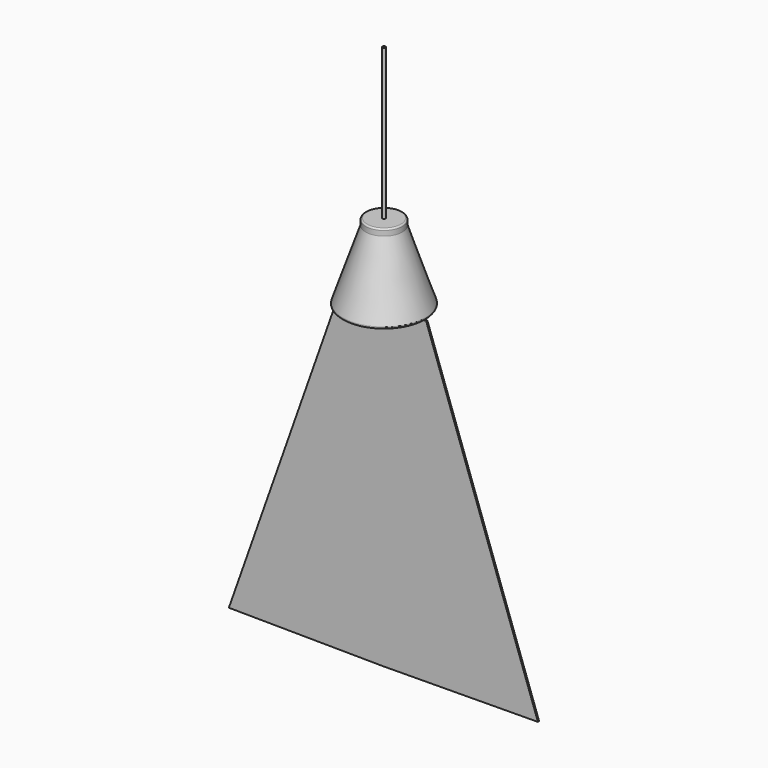
from build123d import *

# Parameters (mm, degrees)
F2_T     = -2
F3_R     = 3
F4_DEPTH = 300
F6_DEPTH = 1.5


# Not quite as in the source:
# - a shell that OpenCascade refuses in one call is made with other operations: the cavity is built on its own and cut out


with BuildPart() as f1:
    # F0 (on Front) → F1 (revolve)
    with BuildSketch(Plane.XZ):
        with BuildLine():
            Line((33.5040265024, 286.039857173), (0, 286.039857173))
            Line((0, 286.039857173), (0, 133.639857173))
            Line((0, 133.639857173), (79.491585897, 133.639857173))
            ThreePointArc((79.491585897, 133.639857173), (81.9292301706, 134.8911746988), (82.33336311, 137.6012635761))
            Line((82.33336311, 137.6012635761), (36.5040265024, 273.0661034584))
            Line((36.5040265024, 273.0661034584), (36.5040265024, 283.039857173))
            ThreePointArc((36.5040265024, 283.039857173), (35.6253468459, 285.1611775165), (33.5040265024, 286.039857173))
        make_face()
    revolve(axis=Axis((0, 0, 248.212441802), (0, 0, 1)))

    # F2: a shell. OpenCascade refuses it in one call, so the cavity is built on its own and cut out:
    # the body offset inwards by the wall thickness, plus a prism from it out through each open face.
    f2_core = offset(f1.part, amount=F2_T, kind=Kind.INTERSECTION, mode=Mode.PRIVATE)
    f2_exits = [f2_core.faces().sort_by_distance(p)[0] for p in [
        (0, 0, 135.639857),
    ]]
    add(f2_core, mode=Mode.SUBTRACT)
    extrude(f2_exits, amount=-F2_T, mode=Mode.SUBTRACT)

    # F3 (on face) → F4 (join)
    with BuildSketch(Plane.XY.offset(286.039857173)):
        Circle(F3_R)
    extrude(amount=F4_DEPTH)

    # F5 (on Front) → F6 (join, symmetric)
    with BuildSketch(Plane.XZ):
        Polygon((85.1287149498, 133.688211441), (0, 133.688211441), (-85.1287149498, 133.688211441), (-307.906627655, -497.1588850021), (0, -499.7738599777), (307.906627655, -497.1588850021), align=None)
    extrude(amount=F6_DEPTH, both=True)


solid = f1.part
